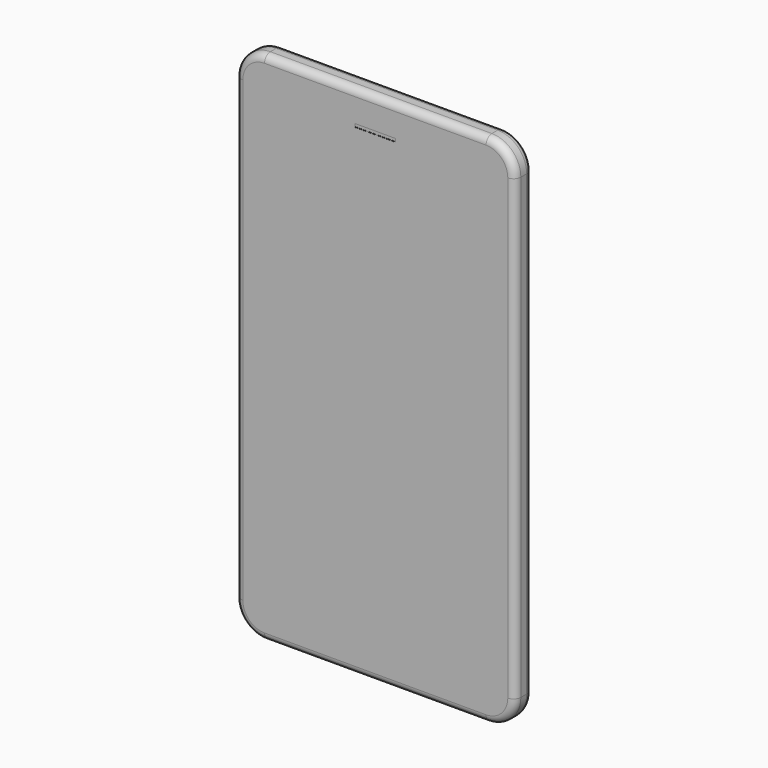
from build123d import *

# Parameters (mm, degrees)
F0_W      = 48.9472970366
F0_H      = 90.3642401099
F1_DEPTH  = 3.81
F2_R      = 5.08
F3_R      = 1.27
F4_R      = 1.27
F7_W      = 7.0798662491
F7_H      = 0.5429834127
F8_DEPTH  = 0.0254
F10_R     = 2.8950348496
F11_DEPTH = 0.381
F12_R     = 0.254


# Not quite as in the source:
# - the program builds the solid bodies; features that only make, move or delete a surface that nothing else refers to are left out


with BuildPart() as f1:
    # F0 (on Front) → F1 (new body)
    with BuildSketch(Plane.XZ):
        Rectangle(F0_W, F0_H)
    extrude(amount=F1_DEPTH)

    # F2
    f2_edges = [f1.edges().sort_by_distance(p)[0] for p in [
        (-24.473649, -1.905, 45.18212),
        (24.473649, -1.905, 45.18212),
        (24.473649, -1.905, -45.18212),
        (-24.473649, -1.905, -45.18212),
    ]]
    fillet(f2_edges, radius=F2_R)

    # F3
    f3_edges = [f1.edges().sort_by_distance(p)[0] for p in [
        (24.473649, 0, 0),
    ]]
    fillet(f3_edges, radius=F3_R)

    # F4
    f4_edges = [f1.edges().sort_by_distance(p)[0] for p in [
        (0, -3.81, 45.18212),
    ]]
    fillet(f4_edges, radius=F4_R)

    # F7 (on face) → F8 (cut)
    with BuildSketch(Plane.XZ.offset(3.81)):
        with Locations((0, 39.5097658038)):
            Rectangle(F7_W, F7_H)
    extrude(amount=-F8_DEPTH, mode=Mode.SUBTRACT)

    # F10 (on face) → F11 (join)
    with BuildSketch(Plane(origin=(0, 0, 0), x_dir=(-1, 0, 0), z_dir=(0, 1, 0))):
        with Locations((-16.5371242911, 39.8641712964)):
            Circle(F10_R)
    extrude(amount=F11_DEPTH)

    # F12
    f12_edges = [f1.edges().sort_by_distance(p)[0] for p in [
        (19.432159, 0.381, 39.864171),
    ]]
    fillet(f12_edges, radius=F12_R)


solid = f1.part
